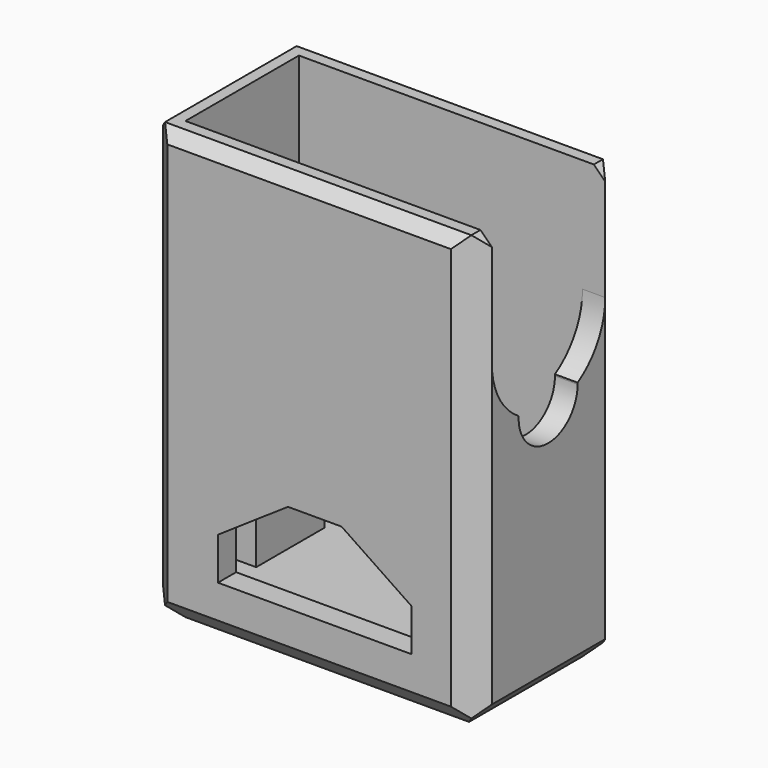
from build123d import *

# Parameters (mm, degrees)
F0_W      = 29
F0_H      = 16.5
F1_DEPTH  = 38.5
F2_T      = -2
F3_DEPTH  = 2.25
F4_SIZE   = 2
F5_SIZE   = 2
F6_SIZE   = 0.99999
F8_DEPTH  = 16.501
F10_DEPTH = 2
F11_R     = 2
F12_DEPTH = 2.001
F13_W     = 7.54
F13_H     = 7.25
F13_R     = 1.1
F14_DEPTH = 4.25


# Not quite as in the source:
# - a fillet or chamfer is up to 0.001 mm smaller than in the source, because OpenCascade refuses the exact size


with BuildPart() as f1:
    # F0 (on Top) → F1 (new body)
    with BuildSketch(Plane.XY):
        with Locations((14.5, 8.25)):
            Rectangle(F0_W, F0_H)
    extrude(amount=F1_DEPTH)

    # F2
    f2_openings = [f1.faces().sort_by_distance(p)[0] for p in [
        (14.5, 8.25, 38.5),
    ]]
    offset(amount=F2_T, openings=f2_openings)

    # F3 (add): a face of the model
    f3_faces = [f1.faces().sort_by_distance(p)[0] for p in [
        (14.5, 8.25, 2),
    ]]
    extrude(f3_faces, amount=F3_DEPTH)

    # F4
    f4_edges = [f1.edges().sort_by_distance(p)[0] for p in [
        (0, 0, 19.25),
        (0, 16.5, 19.25),
        (29, 16.5, 19.25),
        (29, 0, 19.25),
    ]]
    chamfer(f4_edges, length=F4_SIZE)

    # F5 (call 1 of 4: OpenCascade refuses the feature's edges together)
    f5_edges = [f1.edges().sort_by_distance(p)[0] for p in [
        (14.5, 16.5, 0),
    ]]
    chamfer(f5_edges, length=F5_SIZE)

    # F5#2 (call 2 of 4)
    f5_2_edges = [f1.edges().sort_by_distance(p)[0] for p in [
        (29, 8.25, 0),
    ]]
    chamfer(f5_2_edges, length=F5_SIZE)

    # F5#3 (call 3 of 4)
    f5_3_edges = [f1.edges().sort_by_distance(p)[0] for p in [
        (14.5, 0, 0),
    ]]
    chamfer(f5_3_edges, length=F5_SIZE)

    # F5#4 (call 4 of 4)
    f5_4_edges = [f1.edges().sort_by_distance(p)[0] for p in [
        (0, 8.25, 0),
    ]]
    chamfer(f5_4_edges, length=F5_SIZE)

    # F6 (size 1 in the source; OpenCascade refuses exactly that, so slightly less here)
    f6_edges = [f1.edges().sort_by_distance(p)[0] for p in [
        (14.5, 16.5, 38.5),
        (0, 8.25, 38.5),
        (14.5, 0, 38.5),
        (29, 8.25, 38.5),
    ]]
    chamfer(f6_edges, length=F6_SIZE)

    # F7 (on face) → F8 (cut, through all)
    with BuildSketch(Plane.XZ):
        Polygon((6.464, 8.664), (6.464, 4.94), (23.536, 4.94), (23.536, 8.664), (17.364, 12.834), (12.635, 12.834), align=None)
    extrude(amount=-F8_DEPTH, mode=Mode.SUBTRACT)

    # F9 (on face) → F10 (cut, through all)
    with BuildSketch(Plane.YZ.offset(29)):
        with BuildLine():
            Line((2, 28.5), (14.5, 28.5))
            ThreePointArc((14.5, 28.5), (8.25, 34.75), (2, 28.5))
        make_face()
        with BuildLine():
            ThreePointArc((11.4572188031, 23.1356503144), (13.6863414867, 25.4163834155), (14.5, 28.5))
            Line((14.5, 28.5), (2, 28.5))
            ThreePointArc((2, 28.5), (2.7914047728, 25.4559503707), (4.9651962066, 23.1828048711))
            ThreePointArc((4.9651962066, 23.1828048711), (8.2336565888, 26.2499142718), (11.4572188031, 23.1356503144))
        make_face()
        with BuildLine():
            ThreePointArc((2, 28.5), (8.25, 34.75), (14.5, 28.5))
            Line((14.5, 28.5), (14.5, 38.5))
            Line((14.5, 38.5), (2, 38.5))
            Line((2, 38.5), (2, 28.5))
        make_face()
        with BuildLine():
            ThreePointArc((11.4600509613, 23), (11.4593428446, 23.0678399383), (11.4572188031, 23.1356503144))
            ThreePointArc((11.4572188031, 23.1356503144), (8.2046045626, 22.2501648618), (4.9651962066, 23.1828048711))
            ThreePointArc((4.9651962066, 23.1828048711), (8.1186123283, 19.751286566), (11.4600509613, 23))
        make_face()
        with BuildLine():
            ThreePointArc((4.9651962066, 23.1828048711), (8.2046045626, 22.2501648618), (11.4572188031, 23.1356503144))
            ThreePointArc((11.4572188031, 23.1356503144), (8.2336565888, 26.2499142718), (4.9651962066, 23.1828048711))
        make_face()
    extrude(amount=-F10_DEPTH, mode=Mode.SUBTRACT)

    # F11 (on face) → F12 (cut, through all)
    with BuildSketch(Plane.YZ.offset(2)):
        with Locations((8.2100509613, 23)):
            Circle(F11_R)
    extrude(amount=-F12_DEPTH, mode=Mode.SUBTRACT)

    # F13 (on face) → F14 (join)
    with BuildSketch(Plane.YZ.offset(2)):
        with Locations((8.25, 7.875)):
            Rectangle(F13_W, F13_H)
        with Locations((8.25, 9)):
            Circle(F13_R, mode=Mode.SUBTRACT)
    extrude(amount=F14_DEPTH)


solid = f1.part
